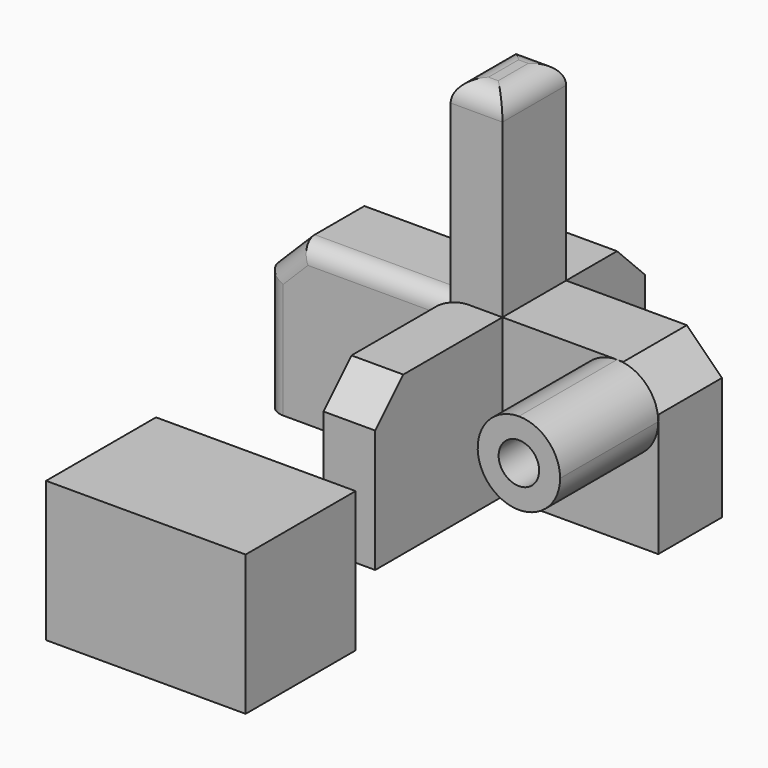
from build123d import *

# Parameters (mm, degrees)
F0_W      = 52.7622997761
F0_H      = 22.692091763
F10_DEPTH = 45
F0_W_2    = 14.7673599422
F0_H_2    = 45.3494936228
F0_W_3    = 44.4295331836
F0_H_3    = 28.1479656696
F2_DEPTH  = 35
F3_SIZE   = 10
F3_2_SIZE = 10
F3_3_SIZE = 10
F3_4_SIZE = 10
F4_W      = 14.7673599422
F4_H      = 22.692091763
F5_DEPTH  = 100
F11_R     = 6
F6_R      = 5.776153979
F7_DEPTH  = 25
F12_R     = 5
F13_R     = 5
F8_W      = 56.9116361439
F8_H      = 39.1838252544
F9_DEPTH  = 40


with BuildPart() as f10:
    # F0 (on Top) → F10 (new body)
    with BuildSketch(Plane.XY):
        with Locations((-26.381149888, 11.3460458815)):
            Rectangle(F0_W, F0_H)
    extrude(amount=F10_DEPTH)

    # F3#4
    f3_4_edges = [f10.edges().sort_by_distance(p)[0] for p in [
        (-52.7623, 11.346046, 45),
    ]]
    chamfer(f3_4_edges, length=F3_4_SIZE)

    # F13
    f13_edges = [f10.edges().sort_by_distance(p)[0] for p in [
        (-47.7623, 0, 40),
        (-21.38115, 0, 45),
        (-52.7623, 0, 17.5),
    ]]
    fillet(f13_edges, radius=F13_R)


with BuildPart() as f10b:
    # F0 (on Top) → F10, piece 2 (new body)
    with BuildSketch(Plane.XY):
        with Locations((7.3836799711, -22.6747468114)):
            Rectangle(F0_W_2, F0_H_2)
    extrude(amount=F10_DEPTH)

    # F3
    f3_edges = [f10b.edges().sort_by_distance(p)[0] for p in [
        (7.38368, -45.349494, 45),
    ]]
    chamfer(f3_edges, length=F3_SIZE)

    # F12
    f12_edges = [f10b.edges().sort_by_distance(p)[0] for p in [
        (0, 0, 22.5),
    ]]
    fillet(f12_edges, radius=F12_R)


with BuildPart() as f10c:
    # F0 (on Top) → F10, piece 3 (new body)
    with BuildSketch(Plane.XY):
        with Locations((36.982126534, 11.3460458815)):
            Rectangle(F0_W_3, F0_H)
    extrude(amount=F10_DEPTH)

    # F3#3
    f3_3_edges = [f10c.edges().sort_by_distance(p)[0] for p in [
        (59.196893, 11.346046, 45),
    ]]
    chamfer(f3_3_edges, length=F3_3_SIZE)


with BuildPart() as f10d:
    # F0 (on Top) → F10, piece 4 (new body)
    with BuildSketch(Plane.XY):
        with Locations((7.3836799711, 36.7660745978)):
            Rectangle(F0_W_2, F0_H_3)
    extrude(amount=F10_DEPTH)

    # F3#2
    f3_2_edges = [f10d.edges().sort_by_distance(p)[0] for p in [
        (7.38368, 50.840057, 45),
    ]]
    chamfer(f3_2_edges, length=F3_2_SIZE)


with BuildPart() as f2:
    # F1 (on face) → F2 (new body)
    with BuildSketch(Plane.XZ):
        with BuildLine():
            ThreePointArc((47.4540758133, 45), (39.1506500614, 24.9537569356), (59.1968931258, 33.2571826875))
            ThreePointArc((59.1968931258, 33.2571826875), (55.7575015652, 41.5606084394), (47.4540758133, 45))
        make_face()
    extrude(amount=F2_DEPTH)

    # F6 (on face) → F7 (cut)
    with BuildSketch(Plane.XZ.offset(35)):
        with Locations((47.4540758133, 33.2571826875)):
            Circle(F6_R)
    extrude(amount=-F7_DEPTH, mode=Mode.SUBTRACT)


with BuildPart() as f5:
    # F4 (on face) → F5 (new body)
    with BuildSketch(Plane.XY):
        with Locations((7.3836799711, 11.3460458815)):
            Rectangle(F4_W, F4_H)
    extrude(amount=F5_DEPTH)

    # F11
    f11_edges = [f5.edges().sort_by_distance(p)[0] for p in [
        (7.38368, 0, 100),
        (14.76736, 11.346046, 100),
        (7.38368, 22.692092, 100),
        (0, 11.346046, 100),
    ]]
    fillet(f11_edges, radius=F11_R)


with BuildPart() as f9:
    # F8 (on Top) → F9 (new body)
    with BuildSketch(Plane.XY):
        with Locations((7.1215014905, -97.9501754045)):
            Rectangle(F8_W, F8_H)
    extrude(amount=F9_DEPTH)


solid = Compound([f10.part, f10b.part, f10c.part, f10d.part, f2.part, f5.part, f9.part])
